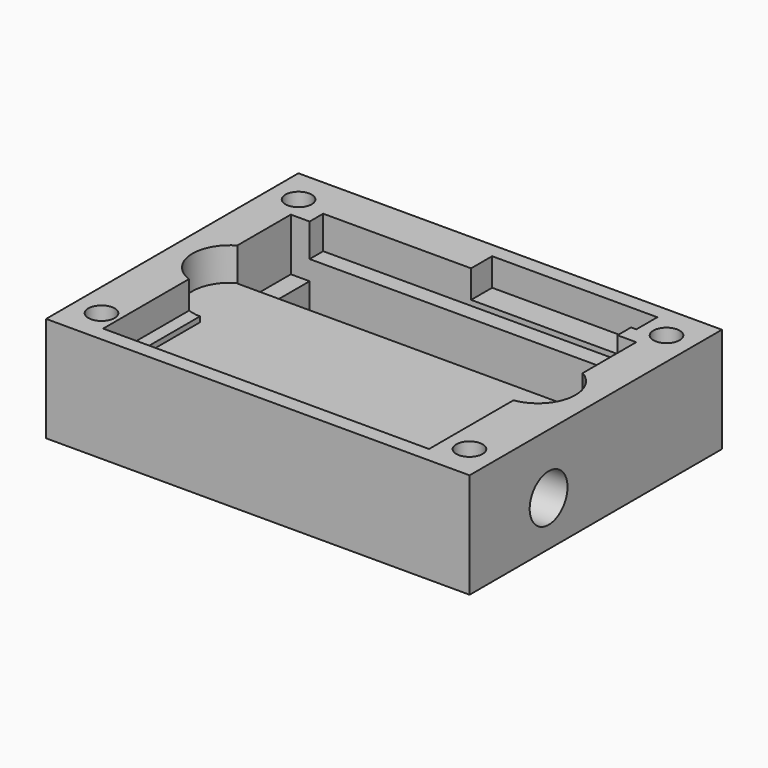
from build123d import *

# Parameters (mm, degrees)
F0_W      = 28.2
F0_H      = 21
F1_DEPTH  = 4
F3_DEPTH  = 2.2
F5_R      = 0.875
F6_DEPTH  = 25
F7_W      = 20.5
F7_H      = 4.5
F8_DEPTH  = 27.5
F9_R      = 1.575
F10_DEPTH = 29
F11_W     = 21
F11_H     = 1
F12_DEPTH = 28.2
F13_W     = 23
F13_H     = 4.5
F14_DEPTH = 3.5
F15_DEPTH = 3
F16_W     = 11
F16_H     = 1.75
F17_DEPTH = 1.85
F18_W     = 21.7
F18_H     = 8
F19_DEPTH = 1.85


# Not quite as in the source:
# - a feature names something its author has since deleted; it is built from what else it names


with BuildPart() as f1:
    # F0 (on Top) → F1 (new body, symmetric)
    with BuildSketch(Plane.XY):
        Rectangle(F0_W, F0_H)
    extrude(amount=F1_DEPTH, both=True)

    # F2 (on face) → F3 (cut)
    with BuildSketch(Plane.XY.offset(4)):
        with BuildLine():
            Line((10.25, 7.75), (-10.25, 7.75))
            Line((-10.25, 7.75), (-10.25, 2.5))
            ThreePointArc((-10.25, 2.5), (-8.482233047, 1.767766953), (-7.75, 0))
            ThreePointArc((-7.75, 0), (-8.482233047, -1.767766953), (-10.25, -2.5))
            Line((-10.25, -2.5), (-10.25, -7.75))
            Line((-10.25, -7.75), (10.25, -7.75))
            Line((10.25, -7.75), (10.25, -2.5))
            ThreePointArc((10.25, -2.5), (7.75, 0), (10.25, 2.5))
            Line((10.25, 2.5), (10.25, 7.75))
        make_face()
        with BuildLine():
            ThreePointArc((-7.75, 0), (-8.482233047, 1.767766953), (-10.25, 2.5))
            Line((-10.25, 2.5), (-10.25, -2.5))
            ThreePointArc((-10.25, -2.5), (-8.482233047, -1.767766953), (-7.75, 0))
        make_face()
        with BuildLine():
            Line((-10.25, -2.5), (-10.25, 2.5))
            ThreePointArc((-10.25, 2.5), (-12.75, 0), (-10.25, -2.5))
        make_face()
        with BuildLine():
            ThreePointArc((12.75, 0), (12.017766953, 1.767766953), (10.25, 2.5))
            Line((10.25, 2.5), (10.25, -2.5))
            ThreePointArc((10.25, -2.5), (12.017766953, -1.767766953), (12.75, 0))
        make_face()
        with BuildLine():
            Line((10.25, -2.5), (10.25, 2.5))
            ThreePointArc((10.25, 2.5), (7.75, 0), (10.25, -2.5))
        make_face()
    extrude(amount=-F3_DEPTH, mode=Mode.SUBTRACT)

    # F5 (on face) → F6 (cut)
    with BuildSketch(Plane.XY.offset(4)):
        with Locations((-12.25, 8.2)):
            Circle(F5_R)
        with Locations((12.25, 8.2)):
            Circle(F5_R)
        with Locations((12.25, -8.2)):
            Circle(F5_R)
        with Locations((-12.25, -8.2)):
            Circle(F5_R)
    extrude(amount=-F6_DEPTH, mode=Mode.SUBTRACT)

    # F7 (on Top) → F8 (cut, symmetric)
    with BuildSketch(Plane.XY):
        with Locations((0, 4.37)):
            Rectangle(F7_W, F7_H)
    extrude(amount=F8_DEPTH, both=True, mode=Mode.SUBTRACT)

    # F9 (on face) → F10 (cut)
    with BuildSketch(Plane.YZ.offset(14.1)):
        with Locations((-3.925, 0)):
            Circle(F9_R)
    extrude(amount=-F10_DEPTH, mode=Mode.SUBTRACT)

    # F11 (on face) → F12 (cut)
    with BuildSketch(Plane.YZ.offset(14.1)):
        with Locations((0, -3.5)):
            Rectangle(F11_W, F11_H)
    extrude(amount=-F12_DEPTH, mode=Mode.SUBTRACT)

    # F13 (on face) → F14 (cut)
    with BuildSketch(Plane.XY.offset(4)):
        with Locations((0, 4.37)):
            Rectangle(F13_W, F13_H)
    extrude(amount=-F14_DEPTH, mode=Mode.SUBTRACT)

    # F13 (on face) → F15 (cut)
    with BuildSketch(Plane.XY.offset(4)):
        with Locations((0, 4.37)):
            Rectangle(F13_W, F13_H)
    extrude(amount=-F15_DEPTH, mode=Mode.SUBTRACT)

    # F16 (on face) → F17 (cut)
    with BuildSketch(Plane.XY.offset(4)):
        with Locations((5.1, 8.625)):
            Rectangle(F16_W, F16_H)
    extrude(amount=-F17_DEPTH, mode=Mode.SUBTRACT)

    # F18 (on face) → F19 (cut)
    with BuildSketch(Plane.XY.offset(4)):
        with Locations((-0.25, -5.5)):
            Rectangle(F18_W, F18_H)
    extrude(amount=-F19_DEPTH, mode=Mode.SUBTRACT)


solid = f1.part
